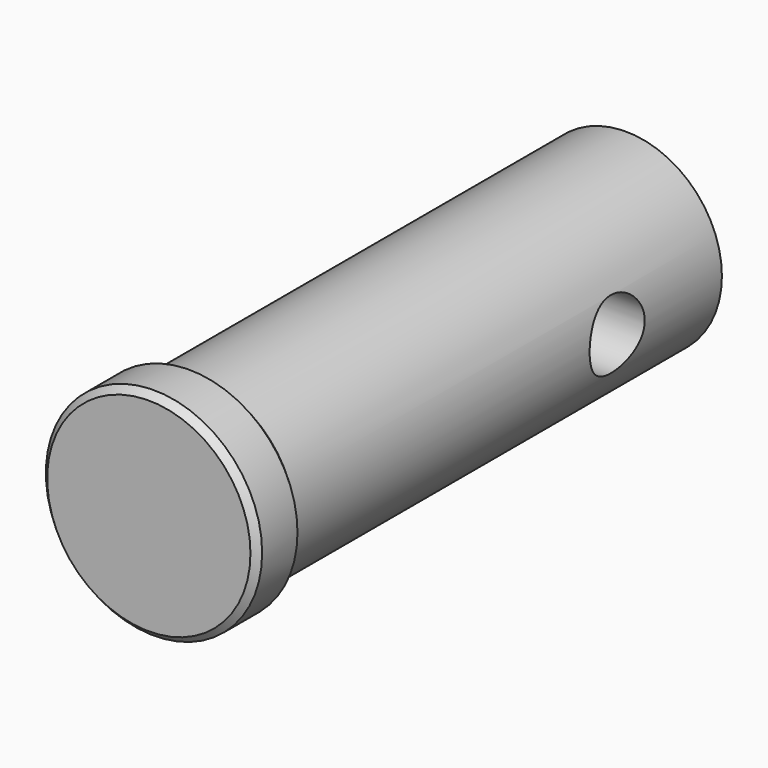
from build123d import *

# Parameters (mm, degrees)
F0_R          = 18.7710767317
F1_DEPTH      = 101.6
F2_R          = 21.1406607176
F3_DEPTH      = 14.986
F4_S5_R       = 18.7710767317
F4_T6_DEPTH   = 32
F5_SIZE2      = 1.27
F5_SIZE       = 1.27
F6_R          = 6.7296542148
F7_DEPTH      = 47.498
F7_DEPTH_BACK = 25.4


# Not quite as in the source:
# - a fillet or chamfer that OpenCascade refuses, or shapes differently, is made with other operations: its cross-section is extruded or revolved along the edge and cut away or added


with BuildPart() as f1:
    # F0 (on Front) → F1 (new body)
    with BuildSketch(Plane.XZ):
        Circle(F0_R)
    extrude(amount=-F1_DEPTH)

    # F2 (on Front) → F3 (join)
    with BuildSketch(Plane.XZ):
        Circle(F2_R)
    extrude(amount=F3_DEPTH)

    # F4: chamfer of 5.08 on 1 edges, made by hand


with BuildPart() as f4_tool2:
    # F4_s3 → F4_t4 (revolve)
    with BuildSketch(Plane.XY):
        Polygon((21.1406607176, -5.08), (16.0606607176, 0), (21.1406607176, 0), align=None)
    revolve(axis=Axis((0, 0, 0), (0, -1, 0)))

    # F4_s5 → F4_t6 (cut, symmetric)
    with BuildSketch(Plane.XZ.offset(2.5)):
        Circle(F4_S5_R)
    extrude(amount=F4_T6_DEPTH, both=True, mode=Mode.SUBTRACT)


with BuildPart() as f1_1:
    add(f1.part)

    # F4_t1: cut F4_tool2
    add(f4_tool2.part, mode=Mode.SUBTRACT)

    # F5
    f5_edges = [f1_1.edges().sort_by_distance(p)[0] for p in [
        (-21.140661, -14.986, 0),
    ]]
    chamfer(f5_edges, length=F5_SIZE, length2=F5_SIZE2)

    # F6 (on Right) → F7 (cut, two sides)
    with BuildSketch(Plane.YZ) as f7_sk:
        with Locations((76.0086998343, 0)):
            Circle(F6_R)
    extrude(amount=F7_DEPTH, mode=Mode.SUBTRACT)
    extrude(f7_sk.sketch, amount=-F7_DEPTH_BACK, mode=Mode.SUBTRACT)


solid = f1_1.part
